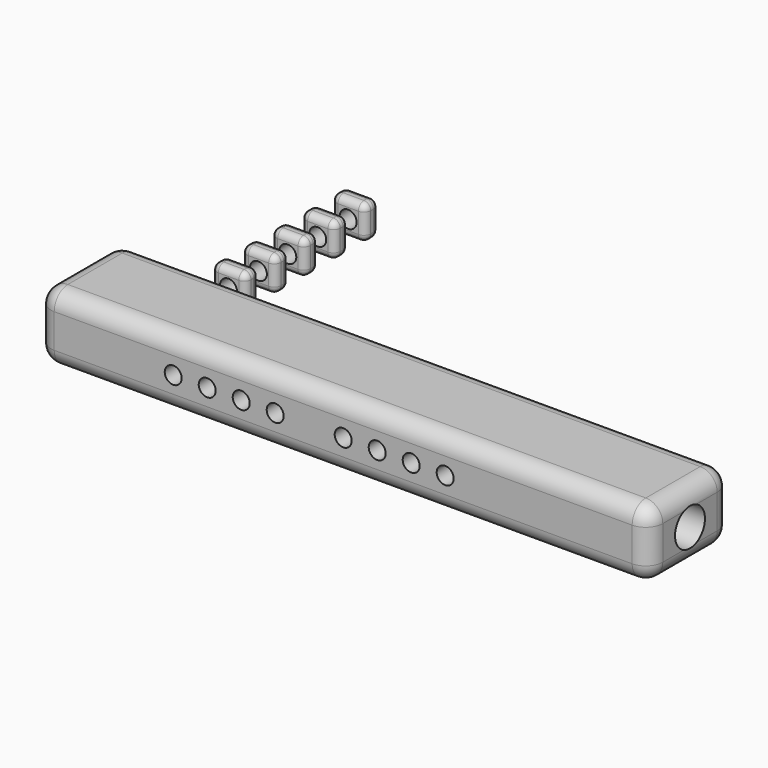
from build123d import *

# Parameters (mm, degrees)
F0_W         = 90
F0_H         = 15
F1_DEPTH     = 10
F2_R         = 2.75
F3_DEPTH     = 90.001
F4_R         = 1.25
F5_DEPTH     = 15.001
F6_T1_DEPTH  = 85
F6_T3_DEPTH  = 10
F6_T5_DEPTH  = 5
F6_S9_W      = 2.5
F6_S9_H      = 2.5
F6_T10_DEPTH = 2.5
F6_S15_W     = 2.5
F6_S15_H     = 2.5
F6_T16_DEPTH = 2.5
F6_S21_W     = 2.5
F6_S21_H     = 2.5
F6_T22_DEPTH = 2.5
F6_S27_W     = 2.5
F6_S27_H     = 2.5
F6_T28_DEPTH = 2.5
F6_S33_W     = 2.5
F6_S33_H     = 2.5
F6_T34_DEPTH = 2.5
F6_S39_W     = 2.5
F6_S39_H     = 2.5
F6_T40_DEPTH = 2.5
F6_S45_W     = 2.5
F6_S45_H     = 2.5
F6_T46_DEPTH = 2.5
F6_S51_W     = 2.5
F6_S51_H     = 2.5
F6_T52_DEPTH = 2.5
F7_W         = 5
F7_H         = 2.5
F8_DEPTH     = 5
F10_R        = 1.25
F11_DEPTH    = 27.0687688377
F12_R        = 1


# Not quite as in the source:
# - a fillet or chamfer that OpenCascade refuses, or shapes differently, is made with other operations: its cross-section is extruded or revolved along the edge and cut away or added


with BuildPart() as f1:
    # F0 (on Top) → F1 (new body)
    with BuildSketch(Plane.XY):
        with Locations((-0.7149035856, 1.6745529257)):
            Rectangle(F0_W, F0_H)
    extrude(amount=F1_DEPTH)

    # F2 (on face) → F3 (cut, through all)
    with BuildSketch(Plane(origin=(-45.7149035856, 0, 0), x_dir=(0, -1, 0), z_dir=(-1, 0, 0))):
        with Locations((-1.6745529257, 5)):
            Circle(F2_R)
    extrude(amount=-F3_DEPTH, mode=Mode.SUBTRACT)

    # F4 (on face) → F5 (cut, through all)
    with BuildSketch(Plane.XZ.offset(5.8254470743)):
        with Locations((-25.714518596, 4.9728379638)):
            Circle(F4_R)
        with Locations((-20.714518596, 4.9728379638)):
            Circle(F4_R)
        with Locations((-15.714518596, 4.9728379638)):
            Circle(F4_R)
        with Locations((-10.7145977698, 4.9447002312)):
            Circle(F4_R)
        with Locations((-0.7149035856, 5)):
            Circle(F4_R)
        with Locations((4.2850915973, 4.9930594514)):
            Circle(F4_R)
        with Locations((9.2850896995, 4.9887031463)):
            Circle(F4_R)
        with Locations((14.2850888268, 4.9857488744)):
            Circle(F4_R)
    extrude(amount=-F5_DEPTH, mode=Mode.SUBTRACT)

    # F6: fillet of radius 2.5 on 12 edges, made by hand

    # F6_s2 → F6_t1 (cut)
    with BuildSketch(Plane.YZ.offset(-43.2149035856)):
        with BuildLine():
            ThreePointArc((9.1745529257, 7.5), (8.4423198787, 9.267766953), (6.6745529257, 10))
            Line((6.6745529257, 10), (9.1745529257, 10))
            Line((9.1745529257, 10), (9.1745529257, 7.5))
        make_face()
        with BuildLine():
            ThreePointArc((-3.3254470743, 10), (-5.0932140272, 9.267766953), (-5.8254470743, 7.5))
            Line((-5.8254470743, 7.5), (-5.8254470743, 10))
            Line((-5.8254470743, 10), (-3.3254470743, 10))
        make_face()
        with BuildLine():
            ThreePointArc((9.1745529257, 2.5), (8.4423198787, 0.732233047), (6.6745529257, 0))
            Line((6.6745529257, 0), (9.1745529257, 0))
            Line((9.1745529257, 0), (9.1745529257, 2.5))
        make_face()
        with BuildLine():
            ThreePointArc((-3.3254470743, 0), (-5.0932140272, 0.732233047), (-5.8254470743, 2.5))
            Line((-5.8254470743, 2.5), (-5.8254470743, 0))
            Line((-5.8254470743, 0), (-3.3254470743, 0))
        make_face()
    extrude(amount=F6_T1_DEPTH, mode=Mode.SUBTRACT)

    # F6_s4 → F6_t3 (cut)
    with BuildSketch(Plane.XZ.offset(-6.6745529257)):
        with BuildLine():
            ThreePointArc((-43.2149035856, 10), (-44.9826705386, 9.267766953), (-45.7149035856, 7.5))
            Line((-45.7149035856, 7.5), (-45.7149035856, 10))
            Line((-45.7149035856, 10), (-43.2149035856, 10))
        make_face()
        with BuildLine():
            ThreePointArc((44.2850964144, 7.5), (43.5528633674, 9.267766953), (41.7850964144, 10))
            Line((41.7850964144, 10), (44.2850964144, 10))
            Line((44.2850964144, 10), (44.2850964144, 7.5))
        make_face()
        with BuildLine():
            ThreePointArc((-43.2149035856, 0), (-44.9826705386, 0.732233047), (-45.7149035856, 2.5))
            Line((-45.7149035856, 2.5), (-45.7149035856, 0))
            Line((-45.7149035856, 0), (-43.2149035856, 0))
        make_face()
        with BuildLine():
            ThreePointArc((44.2850964144, 2.5), (43.5528633674, 0.732233047), (41.7850964144, 0))
            Line((41.7850964144, 0), (44.2850964144, 0))
            Line((44.2850964144, 0), (44.2850964144, 2.5))
        make_face()
    extrude(amount=F6_T3_DEPTH, mode=Mode.SUBTRACT)

    # F6_s6 → F6_t5 (cut)
    with BuildSketch(Plane.XY.offset(2.5)):
        with BuildLine():
            ThreePointArc((41.7850964144, 9.1745529257), (43.5528633674, 8.4423198787), (44.2850964144, 6.6745529257))
            Line((44.2850964144, 6.6745529257), (44.2850964144, 9.1745529257))
            Line((44.2850964144, 9.1745529257), (41.7850964144, 9.1745529257))
        make_face()
        with BuildLine():
            ThreePointArc((44.2850964144, -3.3254470743), (43.5528633674, -5.0932140272), (41.7850964144, -5.8254470743))
            Line((41.7850964144, -5.8254470743), (44.2850964144, -5.8254470743))
            Line((44.2850964144, -5.8254470743), (44.2850964144, -3.3254470743))
        make_face()
        with BuildLine():
            ThreePointArc((-45.7149035856, -3.3254470743), (-44.9826705386, -5.0932140272), (-43.2149035856, -5.8254470743))
            Line((-43.2149035856, -5.8254470743), (-45.7149035856, -5.8254470743))
            Line((-45.7149035856, -5.8254470743), (-45.7149035856, -3.3254470743))
        make_face()
        with BuildLine():
            ThreePointArc((-43.2149035856, 9.1745529257), (-44.9826705386, 8.4423198787), (-45.7149035856, 6.6745529257))
            Line((-45.7149035856, 6.6745529257), (-45.7149035856, 9.1745529257))
            Line((-45.7149035856, 9.1745529257), (-43.2149035856, 9.1745529257))
        make_face()
    extrude(amount=F6_T5_DEPTH, mode=Mode.SUBTRACT)


with BuildPart() as f6_tool8:
    # F6_s9 → F6_t10 (new body)
    with BuildSketch(Plane.XZ.offset(-6.6745529257)):
        with Locations((43.0350964144, 8.75)):
            Rectangle(F6_S9_W, F6_S9_H)
    extrude(amount=-F6_T10_DEPTH)

    # F6_s11 → F6_t12 (revolve, cut)
    with BuildSketch(Plane(origin=(41.7850964144, 6.6745529257, 7.5), x_dir=(-0.7071067812, 0, -0.7071067812), z_dir=(0.7071067812, 0, -0.7071067812))):
        with BuildLine():
            ThreePointArc((0, -2.5), (2.5, 0), (0, 2.5))
            Line((0, 2.5), (0, -2.5))
        make_face()
    revolve(axis=Axis((41.7850964144, 6.6745529257, 7.5), (0, 1, 0)), mode=Mode.SUBTRACT)


with BuildPart() as f1_1:
    add(f1.part)

    # F6_t7: cut F6_tool8
    add(f6_tool8.part, mode=Mode.SUBTRACT)


with BuildPart() as f6_tool14:
    # F6_s15 → F6_t16 (new body)
    with BuildSketch(Plane.XZ.offset(-6.6745529257)):
        with Locations((-44.4649035856, 8.75)):
            Rectangle(F6_S15_W, F6_S15_H)
    extrude(amount=-F6_T16_DEPTH)

    # F6_s17 → F6_t18 (revolve, cut)
    with BuildSketch(Plane(origin=(-43.2149035856, 6.6745529257, 7.5), x_dir=(0.7071067812, 0, -0.7071067812), z_dir=(0.7071067812, 0, 0.7071067812))):
        with BuildLine():
            ThreePointArc((0, -2.5), (2.5, 0), (0, 2.5))
            Line((0, 2.5), (0, -2.5))
        make_face()
    revolve(axis=Axis((-43.2149035856, 6.6745529257, 7.5), (0, 1, 0)), mode=Mode.SUBTRACT)


with BuildPart() as f1_2:
    add(f1_1.part)

    # F6_t13: cut F6_tool14
    add(f6_tool14.part, mode=Mode.SUBTRACT)


with BuildPart() as f6_tool20:
    # F6_s21 → F6_t22 (new body)
    with BuildSketch(Plane.XY.offset(7.5)):
        with Locations((-44.4649035856, -4.5754470743)):
            Rectangle(F6_S21_W, F6_S21_H)
    extrude(amount=F6_T22_DEPTH)

    # F6_s23 → F6_t24 (revolve, cut)
    with BuildSketch(Plane(origin=(-43.2149035856, -3.3254470743, 7.5), x_dir=(0.7071067812, 0.7071067812, 0), z_dir=(0.7071067812, -0.7071067812, 0))):
        with BuildLine():
            ThreePointArc((0, -2.5), (2.5, 0), (0, 2.5))
            Line((0, 2.5), (0, -2.5))
        make_face()
    revolve(axis=Axis((-43.2149035856, -3.3254470743, 7.5), (0, 0, 1)), mode=Mode.SUBTRACT)


with BuildPart() as f1_3:
    add(f1_2.part)

    # F6_t19: cut F6_tool20
    add(f6_tool20.part, mode=Mode.SUBTRACT)


with BuildPart() as f6_tool26:
    # F6_s27 → F6_t28 (new body)
    with BuildSketch(Plane.YZ.offset(41.7850964144)):
        with Locations((-4.5754470743, 8.75)):
            Rectangle(F6_S27_W, F6_S27_H)
    extrude(amount=F6_T28_DEPTH)

    # F6_s29 → F6_t30 (revolve, cut)
    with BuildSketch(Plane(origin=(41.7850964144, -3.3254470743, 7.5), x_dir=(0, 0.7071067812, -0.7071067812), z_dir=(0, -0.7071067812, -0.7071067812))):
        with BuildLine():
            ThreePointArc((0, -2.5), (2.5, 0), (0, 2.5))
            Line((0, 2.5), (0, -2.5))
        make_face()
    revolve(axis=Axis((41.7850964144, -3.3254470743, 7.5), (1, 0, 0)), mode=Mode.SUBTRACT)


with BuildPart() as f1_4:
    add(f1_3.part)

    # F6_t25: cut F6_tool26
    add(f6_tool26.part, mode=Mode.SUBTRACT)


with BuildPart() as f6_tool32:
    # F6_s33 → F6_t34 (new body)
    with BuildSketch(Plane.XZ.offset(-6.6745529257)):
        with Locations((43.0350964144, 1.25)):
            Rectangle(F6_S33_W, F6_S33_H)
    extrude(amount=-F6_T34_DEPTH)

    # F6_s35 → F6_t36 (revolve, cut)
    with BuildSketch(Plane(origin=(41.7850964144, 6.6745529257, 2.5), x_dir=(-0.7071067812, 0, 0.7071067812), z_dir=(-0.7071067812, 0, -0.7071067812))):
        with BuildLine():
            ThreePointArc((0, -2.5), (2.5, 0), (0, 2.5))
            Line((0, 2.5), (0, -2.5))
        make_face()
    revolve(axis=Axis((41.7850964144, 6.6745529257, 2.5), (0, 1, 0)), mode=Mode.SUBTRACT)


with BuildPart() as f1_5:
    add(f1_4.part)

    # F6_t31: cut F6_tool32
    add(f6_tool32.part, mode=Mode.SUBTRACT)


with BuildPart() as f6_tool38:
    # F6_s39 → F6_t40 (new body)
    with BuildSketch(Plane.XZ.offset(-6.6745529257)):
        with Locations((-44.4649035856, 1.25)):
            Rectangle(F6_S39_W, F6_S39_H)
    extrude(amount=-F6_T40_DEPTH)

    # F6_s41 → F6_t42 (revolve, cut)
    with BuildSketch(Plane(origin=(-43.2149035856, 6.6745529257, 2.5), x_dir=(0.7071067812, 0, 0.7071067812), z_dir=(-0.7071067812, 0, 0.7071067812))):
        with BuildLine():
            ThreePointArc((0, -2.5), (2.5, 0), (0, 2.5))
            Line((0, 2.5), (0, -2.5))
        make_face()
    revolve(axis=Axis((-43.2149035856, 6.6745529257, 2.5), (0, 1, 0)), mode=Mode.SUBTRACT)


with BuildPart() as f1_6:
    add(f1_5.part)

    # F6_t37: cut F6_tool38
    add(f6_tool38.part, mode=Mode.SUBTRACT)


with BuildPart() as f6_tool44:
    # F6_s45 → F6_t46 (new body)
    with BuildSketch(Plane.XY.offset(2.5)):
        with Locations((-44.4649035856, -4.5754470743)):
            Rectangle(F6_S45_W, F6_S45_H)
    extrude(amount=-F6_T46_DEPTH)

    # F6_s47 → F6_t48 (revolve, cut)
    with BuildSketch(Plane(origin=(-43.2149035856, -3.3254470743, 2.5), x_dir=(0.7071067812, 0.7071067812, 0), z_dir=(-0.7071067812, 0.7071067812, 0))):
        with BuildLine():
            ThreePointArc((0, -2.5), (2.5, 0), (0, 2.5))
            Line((0, 2.5), (0, -2.5))
        make_face()
    revolve(axis=Axis((-43.2149035856, -3.3254470743, 2.5), (0, 0, -1)), mode=Mode.SUBTRACT)


with BuildPart() as f1_7:
    add(f1_6.part)

    # F6_t43: cut F6_tool44
    add(f6_tool44.part, mode=Mode.SUBTRACT)


with BuildPart() as f6_tool50:
    # F6_s51 → F6_t52 (new body)
    with BuildSketch(Plane.YZ.offset(41.7850964144)):
        with Locations((-4.5754470743, 1.25)):
            Rectangle(F6_S51_W, F6_S51_H)
    extrude(amount=F6_T52_DEPTH)

    # F6_s53 → F6_t54 (revolve, cut)
    with BuildSketch(Plane(origin=(41.7850964144, -3.3254470743, 2.5), x_dir=(0, 0.7071067812, 0.7071067812), z_dir=(0, 0.7071067812, -0.7071067812))):
        with BuildLine():
            ThreePointArc((0, -2.5), (2.5, 0), (0, 2.5))
            Line((0, 2.5), (0, -2.5))
        make_face()
    revolve(axis=Axis((41.7850964144, -3.3254470743, 2.5), (1, 0, 0)), mode=Mode.SUBTRACT)


with BuildPart() as f1_8:
    add(f1_7.part)

    # F6_t49: cut F6_tool50
    add(f6_tool50.part, mode=Mode.SUBTRACT)


with BuildPart() as f8:
    # F7 (on Top) → F8 (new body)
    with BuildSketch(Plane.XY):
        with Locations((-37.2249409556, 19.9923216634)):
            Rectangle(F7_W, F7_H)
    extrude(amount=F8_DEPTH)

    # F10 (on face) → F11 (cut, through all)
    with BuildSketch(Plane(origin=(0, 21.2423216634, 0), x_dir=(-1, 0, 0), z_dir=(0, 1, 0))):
        with Locations((37.240523845, 2.479522489)):
            Circle(F10_R)
    extrude(amount=-F11_DEPTH, mode=Mode.SUBTRACT)

    # F12
    f12_edges = [f8.edges().sort_by_distance(p)[0] for p in [
        (-37.224941, 21.242322, 5),
        (-39.724941, 19.992322, 5),
        (-37.224941, 18.742322, 5),
        (-34.724941, 19.992322, 5),
        (-39.724941, 21.242322, 2.5),
        (-39.724941, 18.742322, 2.5),
        (-39.724941, 19.992322, 0),
        (-37.224941, 21.242322, 0),
        (-37.224941, 18.742322, 0),
        (-34.724941, 19.992322, 0),
        (-34.724941, 18.742322, 2.5),
        (-34.724941, 21.242322, 2.5),
    ]]
    fillet(f12_edges, radius=F12_R)


with BuildPart() as f13_1:
    # F13: copy of F8
    add(f8.part)


with BuildPart() as f15_1:
    # F15: copy of F13_1
    add(f13_1.part.moved(Location((0, 5.5, 0))))


with BuildPart() as f16_1:
    # F16: copy of F15_1
    add(f15_1.part.moved(Location((0, 5.4, 0))))


with BuildPart() as f17_1:
    # F17: copy of F16_1
    add(f16_1.part.moved(Location((0, 5.5, 0))))


with BuildPart() as f18_1:
    # F18: copy of F17_1
    add(f17_1.part.moved(Location((0, 5.6, 0))))


solid = Compound([f1_8.part, f13_1.part, f15_1.part, f16_1.part, f17_1.part, f18_1.part])
